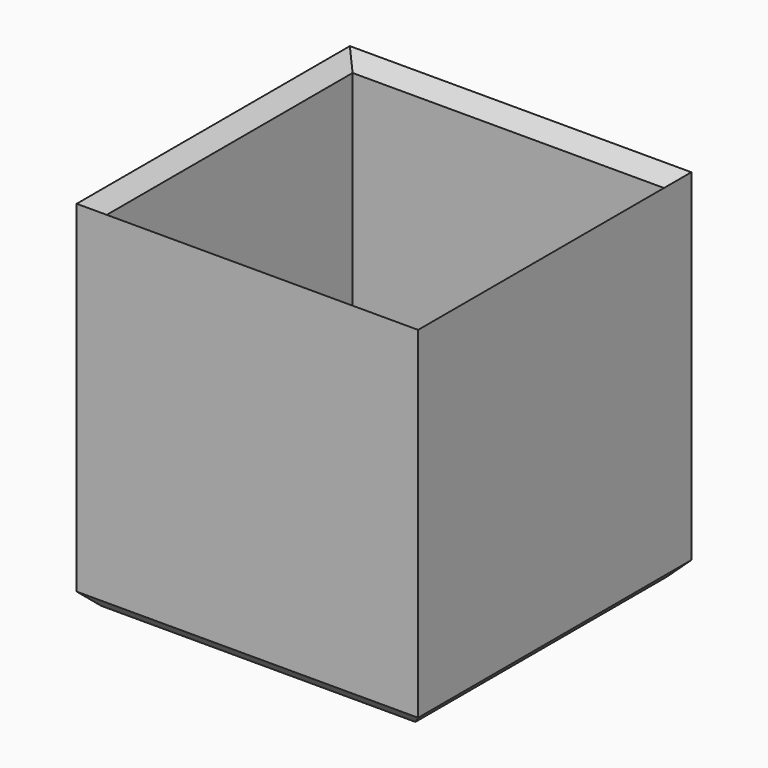
from build123d import *

# Parameters (mm, degrees)
F0_W     = 50
F0_H     = 50
F0_W_2   = 46
F0_H_2   = 46
F1_DEPTH = 50
F2_DEPTH = 2
F3_SIZE  = 1.99999


# Not quite as in the source:
# - a fillet or chamfer is up to 0.001 mm smaller than in the source, because OpenCascade refuses the exact size


with BuildPart() as f1:
    # F0 (on Top) → F1 (new body)
    with BuildSketch(Plane.XY):
        Rectangle(F0_W, F0_H)
        Rectangle(F0_W_2, F0_H_2, mode=Mode.SUBTRACT)
    extrude(amount=F1_DEPTH)

    # F0 (on Top) → F2 (join)
    with BuildSketch(Plane.XY):
        Rectangle(F0_W, F0_H)
        Rectangle(F0_W_2, F0_H_2, mode=Mode.SUBTRACT)
        Rectangle(F0_W_2, F0_H_2)
    extrude(amount=-F2_DEPTH)

    # F3 (size 2 in the source; OpenCascade refuses exactly that, so slightly less here)
    f3_edges = [f1.edges().sort_by_distance(p)[0] for p in [
        (0, -25, -2),
        (-25, 0, -2),
        (25, 0, -2),
        (0, 25, -2),
        (-23, 0, 50),
        (0, 23, 50),
        (23, 0, 50),
        (0, -23, 50),
    ]]
    chamfer(f3_edges, length=F3_SIZE)


solid = f1.part
